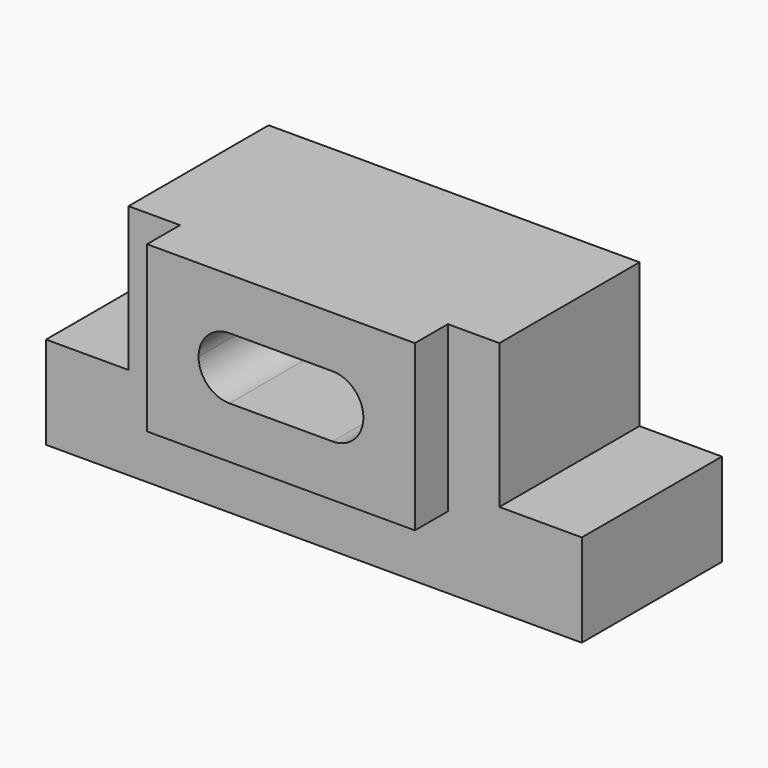
from build123d import *

# Parameters (mm, degrees)
F0_W     = 18
F0_H     = 7
F1_DEPTH = 4.25
F2_W     = 13
F2_H     = 8
F3_DEPTH = 2
F4_W     = 8
F4_H     = 3
F5_DEPTH = 10.5
F6_R     = 1.49999


# Not quite as in the source:
# - a fillet or chamfer is up to 0.001 mm smaller than in the source, because OpenCascade refuses the exact size


with BuildPart() as f1:
    # F0 (on Front) → F1 (new body, symmetric)
    with BuildSketch(Plane.XZ):
        Polygon((-13, 4.5), (-13, 0), (13, 0), (13, 4.5), (9, 4.5), (-9, 4.5), align=None)
        with Locations((0, 8)):
            Rectangle(F0_W, F0_H)
    extrude(amount=F1_DEPTH, both=True)

    # F2 (on face) → F3 (join)
    with BuildSketch(Plane.XZ.offset(4.25)):
        with Locations((0, 7.5)):
            Rectangle(F2_W, F2_H)
    extrude(amount=F3_DEPTH)

    # F4 (on face) → F5 (cut, through all)
    with BuildSketch(Plane.XZ.offset(6.25)):
        with Locations((0, 7.5)):
            Rectangle(F4_W, F4_H)
    extrude(amount=-F5_DEPTH, mode=Mode.SUBTRACT)

    # F6 (radius 1.5 in the source; OpenCascade refuses exactly that, so slightly less here)
    f6_edges = [f1.edges().sort_by_distance(p)[0] for p in [
        (-4, -1, 6),
        (-4, -1, 9),
        (4, -1, 6),
        (4, -1, 9),
    ]]
    fillet(f6_edges, radius=F6_R)


solid = f1.part
